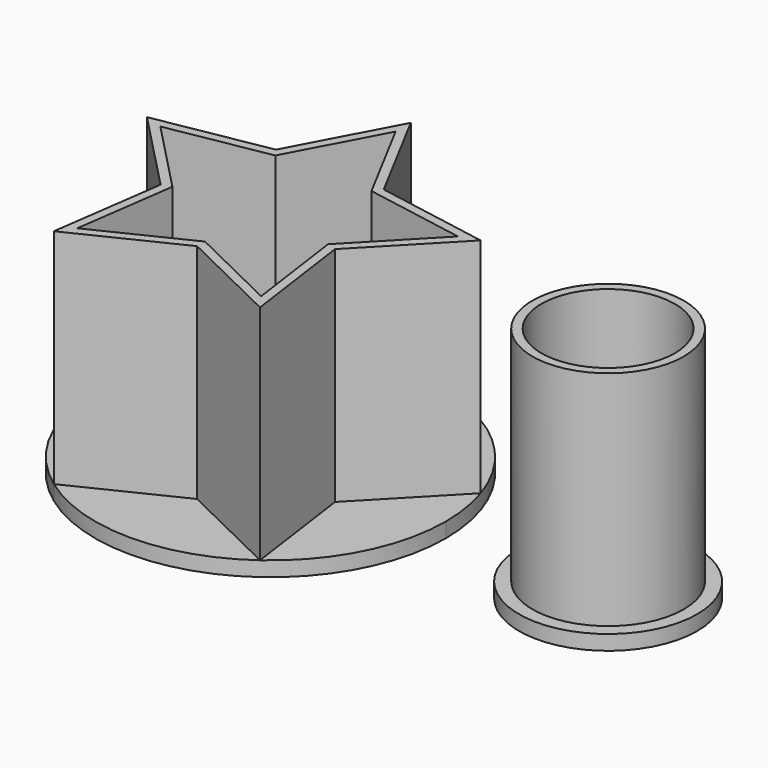
from build123d import *

# Parameters (mm, degrees)
F0_R     = 5.1
F0_R_2   = 4.5
F1_DEPTH = 15
F0_R_3   = 6
F0_R_4   = 3.5
F2_DEPTH = 1
F4_DEPTH = 15
F5_T     = -0.6
F6_DEPTH = 25
F8_DEPTH = 1


# Not quite as in the source:
# - a feature names something its author has since deleted; it is built from what else it names


with BuildPart() as f1:
    # F0 (on Top) → F1 (new body)
    with BuildSketch(Plane.XY):
        Circle(F0_R)
        Circle(F0_R_2, mode=Mode.SUBTRACT)
    extrude(amount=F1_DEPTH)

    # F0 (on Top) → F2 (join)
    with BuildSketch(Plane.XY):
        Circle(F0_R_3)
        Circle(F0_R, mode=Mode.SUBTRACT)
        Circle(F0_R)
        Circle(F0_R_2, mode=Mode.SUBTRACT)
        Circle(F0_R_2)
        Circle(F0_R_4, mode=Mode.SUBTRACT)
    extrude(amount=-F2_DEPTH)


with BuildPart() as f4:
    # F3 (on Top) → F4 (new body)
    with BuildSketch(Plane.XY):
        Polygon((-22.7533387916, 11.8196601125), (-26.3860514316, 5), (-19.1206261516, 5), align=None)
        Polygon((-19.1206261516, 5), (-26.3860514316, 5), (-28.6311913145, -1.9098300563), (-22.7533387916, -6.1803398875), (-16.8754862687, -1.9098300563), align=None)
        Polygon((-28.6311913145, -1.9098300563), (-26.3860514316, 5), (-33.9944407131, 3.6526692678), align=None)
        Polygon((-11.5122368701, 3.6526692679), (-19.1206261516, 5), (-16.8754862687, -1.9098300563), align=None)
        Polygon((-22.7533387916, -6.1803398875), (-28.6311913145, -1.9098300563), (-29.7009252298, -9.5621863542), align=None)
        Polygon((-15.8057523534, -9.5621863542), (-16.8754862687, -1.9098300563), (-22.7533387916, -6.1803398875), align=None)
    extrude(amount=F4_DEPTH)

    # F5
    f5_openings = [f4.faces().sort_by_distance(p)[0] for p in [
        (-22.753339, 2.4e-05, 15),
    ]]
    offset(amount=F5_T, openings=f5_openings, kind=Kind.INTERSECTION)

    # F6 (cut): a face of the model
    f6_faces = [f4.faces().sort_by_distance(p)[0] for p in [
        (-22.7533387916, 1.8747e-05, 0.6),
    ]]
    extrude(f6_faces, amount=-F6_DEPTH, mode=Mode.SUBTRACT)

    # F7 (on face) → F8 (join)
    with BuildSketch(Plane(origin=(0, 0, 0), x_dir=(1, 0, 0), z_dir=(0, 0, -1))):
        with BuildLine():
            ThreePointArc((-33.9937850005, -3.6527853846), (-20.9025615121, -11.6750787208), (-10.931109278, 0))
            ThreePointArc((-10.931109278, 0), (-17.3859492082, 10.5325851378), (-29.7009252298, 9.5621863542))
            Line((-29.7009252298, 9.5621863542), (-22.7533387916, 6.1803398875))
            Line((-22.7533387916, 6.1803398875), (-15.8057523534, 9.5621863542))
            Line((-15.8057523534, 9.5621863542), (-16.8753003708, 1.9111598792))
            ThreePointArc((-16.8753003708, 1.9111598792), (-16.8749270082, 1.9100114851), (-16.87455387, 1.9088630181))
            Line((-16.87455387, 1.9088630181), (-11.5122368701, -3.6526692679))
            Line((-11.5122368701, -3.6526692679), (-19.1206261516, -5))
            Line((-19.1206261516, -5), (-22.7533387916, -11.8196601125))
            Line((-22.7533387916, -11.8196601125), (-26.3860514316, -5))
            Line((-26.3860514316, -5), (-33.9937850005, -3.6527853846))
        make_face()
        with BuildLine():
            Line((-28.6311913145, 1.9098300563), (-29.7009252298, 9.5621863542))
            ThreePointArc((-29.7009252298, 9.5621863542), (-33.9939295406, 3.6523405078), (-33.9939784806, -3.652189863))
            Line((-33.9939784806, -3.652189863), (-28.6311913145, 1.9098300563))
        make_face()
        with BuildLine():
            Line((-22.7533387916, 6.1803398875), (-29.7009252298, 9.5621863542))
            Line((-29.7009252298, 9.5621863542), (-28.6311913145, 1.9098300563))
            Line((-28.6311913145, 1.9098300563), (-33.9939784806, -3.652189863))
            ThreePointArc((-33.9939784806, -3.652189863), (-33.9938817445, -3.6524876251), (-33.9937850005, -3.6527853846))
            Line((-33.9937850005, -3.6527853846), (-26.3860514316, -5))
            Line((-26.3860514316, -5), (-22.7533387916, -11.8196601125))
            Line((-22.7533387916, -11.8196601125), (-19.1206261516, -5))
            ThreePointArc((-19.1206261516, -5), (-19.6033787354, -5.3172164164), (-20.1136429421, -5.587968612))
            Line((-20.1136429421, -5.587968612), (-22.7533387916, -10.5434468668))
            Line((-22.7533387916, -10.5434468668), (-25.3941234048, -5.5859246852))
            ThreePointArc((-25.3941234048, -5.5859246852), (-26.3846353663, -4.9986775768), (-27.2489939544, -4.2378508268))
            Line((-27.2489939544, -4.2378508268), (-32.780698951, -3.25826949))
            Line((-32.780698951, -3.25826949), (-28.8808590942, 0.7864532062))
            ThreePointArc((-28.8808590942, 0.7864532062), (-28.6287938191, 1.9091510398), (-28.1729521499, 2.9656526731))
            Line((-28.1729521499, 2.9656526731), (-28.9507619198, 8.5297255762))
            Line((-28.9507619198, 8.5297255762), (-23.9008499041, 6.0716018437))
            ThreePointArc((-23.9008499041, 6.0716018437), (-22.7529067543, 6.1793887762), (-21.6049223097, 6.0720425464))
            Line((-21.6049223097, 6.0720425464), (-16.5559156634, 8.5297255762))
            Line((-16.5559156634, 8.5297255762), (-17.333067283, 2.9703607601))
            ThreePointArc((-17.333067283, 2.9703607601), (-17.0794064137, 2.4514686566), (-16.8753003708, 1.9111598792))
            Line((-16.8753003708, 1.9111598792), (-15.8057523534, 9.5621863542))
            Line((-15.8057523534, 9.5621863542), (-22.7533387916, 6.1803398875))
        make_face()
        with BuildLine():
            Line((-16.8754862687, 1.9098300563), (-16.8753003708, 1.9111598792))
            ThreePointArc((-16.8753003708, 1.9111598792), (-17.0794064137, 2.4514686566), (-17.333067283, 2.9703607601))
            Line((-17.333067283, 2.9703607601), (-17.5101449471, 1.7036332513))
            Line((-17.5101449471, 1.7036332513), (-16.6220867723, 0.7825828526))
            ThreePointArc((-16.6220867723, 0.7825828526), (-16.7219659069, 1.351630544), (-16.87455387, 1.9088630181))
            Line((-16.87455387, 1.9088630181), (-16.8754862687, 1.9098300563))
        make_face()
        with BuildLine():
            ThreePointArc((-20.1136429421, -5.587968612), (-19.6033787354, -5.3172164164), (-19.1206261516, -5))
            ThreePointArc((-19.1206261516, -5), (-18.6693555038, -4.6388729337), (-18.2537991943, -4.2371629522))
            Line((-18.2537991943, -4.2371629522), (-19.5128597724, -4.4601235484))
            Line((-19.5128597724, -4.4601235484), (-20.1136429421, -5.587968612))
        make_face()
        with BuildLine():
            ThreePointArc((-18.2537991943, -4.2371629522), (-18.6693555038, -4.6388729337), (-19.1206261516, -5))
            Line((-19.1206261516, -5), (-11.5122368701, -3.6526692679))
            Line((-11.5122368701, -3.6526692679), (-16.87455387, 1.9088630181))
            ThreePointArc((-16.87455387, 1.9088630181), (-16.7219659069, 1.351630544), (-16.6220867723, 0.7825828526))
            Line((-16.6220867723, 0.7825828526), (-12.7259786322, -3.2582694901))
            Line((-12.7259786322, -3.2582694901), (-18.2537991943, -4.2371629522))
        make_face()
        with BuildLine():
            ThreePointArc((-21.6049223097, 6.0720425464), (-19.1211013467, 5.0003450612), (-17.333067283, 2.9703607601))
            Line((-17.333067283, 2.9703607601), (-16.5559156634, 8.5297255762))
            Line((-16.5559156634, 8.5297255762), (-21.6049223097, 6.0720425464))
        make_face()
        with BuildLine():
            Line((-22.7533387916, -10.5434468668), (-20.1136429421, -5.587968612))
            ThreePointArc((-20.1136429421, -5.587968612), (-22.7541124911, -6.1793884271), (-25.3941234048, -5.5859246852))
            Line((-25.3941234048, -5.5859246852), (-22.7533387916, -10.5434468668))
        make_face()
        with BuildLine():
            ThreePointArc((-16.5723317321, 0), (-17.0080609546, -2.2793026735), (-18.2537991943, -4.2371629522))
            Line((-18.2537991943, -4.2371629522), (-12.7259786322, -3.2582694901))
            Line((-12.7259786322, -3.2582694901), (-16.6220867723, 0.7825828526))
            ThreePointArc((-16.6220867723, 0.7825828526), (-16.5847830367, 0.39208146), (-16.5723317321, 0))
        make_face()
        with BuildLine():
            Line((-22.7533387916, 5.5130328448), (-21.6049223097, 6.0720425464))
            ThreePointArc((-21.6049223097, 6.0720425464), (-22.7529067543, 6.1793887762), (-23.9008499041, 6.0716018437))
            Line((-23.9008499041, 6.0716018437), (-22.7533387916, 5.5130328448))
        make_face()
        with BuildLine():
            ThreePointArc((-27.2489939544, -4.2378508268), (-26.3846353663, -4.9986775768), (-25.3941234048, -5.5859246852))
            Line((-25.3941234048, -5.5859246852), (-25.9938178107, -4.4601235484))
            Line((-25.9938178107, -4.4601235484), (-27.2489939544, -4.2378508268))
        make_face()
        with BuildLine():
            ThreePointArc((-28.1729521499, 2.9656526731), (-26.3854708, 4.9980702976), (-23.9008499041, 6.0716018437))
            Line((-23.9008499041, 6.0716018437), (-28.9507619198, 8.5297255762))
            Line((-28.9507619198, 8.5297255762), (-28.1729521499, 2.9656526731))
        make_face()
        with BuildLine():
            Line((-32.780698951, -3.25826949), (-27.2489939544, -4.2378508268))
            ThreePointArc((-27.2489939544, -4.2378508268), (-28.6288853053, -1.9088693886), (-28.8808590942, 0.7864532062))
            Line((-28.8808590942, 0.7864532062), (-32.780698951, -3.25826949))
        make_face()
        with BuildLine():
            Line((-27.9965326361, 1.7036332513), (-28.1729521499, 2.9656526731))
            ThreePointArc((-28.1729521499, 2.9656526731), (-28.6287938191, 1.9091510398), (-28.8808590942, 0.7864532062))
            Line((-28.8808590942, 0.7864532062), (-27.9965326361, 1.7036332513))
        make_face()
    extrude(amount=F8_DEPTH)


solid = Compound([f1.part, f4.part])
